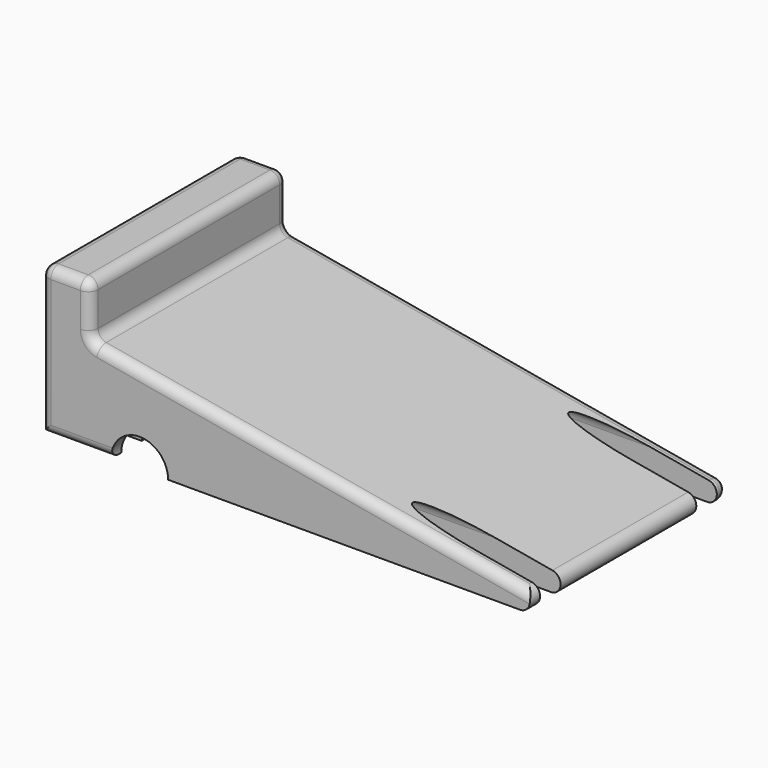
from build123d import *

# Parameters (mm, degrees)
F1_DEPTH = 15.875
F3_DEPTH = 76.201
F5_DEPTH = 31.751
F6_F1_R  = 1.27
F6_F2_R  = 1.27


with BuildPart() as f1:
    # F0 (on Front) → F1 (new body, symmetric)
    with BuildSketch(Plane.XZ):
        Polygon((-38.1, 19.05), (-38.1, 0), (38.1, 0), (-31.75, 12.3164396025), (-31.75, 19.05), align=None)
    extrude(amount=F1_DEPTH, both=True)

    # F2 (on face) → F3 (cut, through all)
    with BuildSketch(Plane(origin=(-38.1, 0, 0), x_dir=(0, -1, 0), z_dir=(-1, 0, 0))):
        with BuildLine():
            Line((-10.922, 0), (-10.922, 3.81))
            ThreePointArc((-10.922, 3.81), (-12.5728756711, 5.4608756711), (-14.2237513422, 3.81))
            Line((-14.2237513422, 3.81), (-14.2237513422, 0))
            Line((-14.2237513422, 0), (-10.922, 0))
        make_face()
        with BuildLine():
            Line((14.2237513422, 0), (14.2237513422, 3.81))
            ThreePointArc((14.2237513422, 3.81), (12.5728756711, 5.4608756711), (10.922, 3.81))
            Line((10.922, 3.81), (10.922, 0))
            Line((10.922, 0), (14.2237513422, 0))
        make_face()
    extrude(amount=-F3_DEPTH, mode=Mode.SUBTRACT)

    # F4 (on face) → F5 (cut, through all)
    with BuildSketch(Plane(origin=(0, 15.875, 0), x_dir=(-1, 0, 0), z_dir=(0, 1, 0))):
        with BuildLine():
            ThreePointArc((29.083, 0), (25.4, 3.683), (21.717, 0))
            Line((21.717, 0), (29.083, 0))
        make_face()
    extrude(amount=-F5_DEPTH, mode=Mode.SUBTRACT)

    # F6: fillet of radius 1.27 on 17 edges, made by hand

    # F6_f1
    f6_f1_edges = [f1.edges().sort_by_distance(p)[0] for p in [
        (-31.75, 0, 12.3164396025),
    ]]
    fillet(f6_f1_edges, radius=F6_F1_R)

    # F6_f2
    f6_f2_edges = [f1.edges().sort_by_distance(p)[0] for p in [
        (38.1, 0, 0),
        (38.1, 15.0493756711, 0),
        (38.1, -15.0493756711, 0),
        (-31.75, 0, 19.05),
        (-38.1, 0, 19.05),
        (-38.1, 15.0493756711, 0),
        (-38.1, 0, 0),
        (-33.5915, -15.875, 0),
        (8.1915, 15.875, 0),
        (-33.5915, 15.875, 0),
        (3.6997334072, -15.875, 6.0656951439),
        (-38.1, -15.875, 9.525),
        (-38.1, 15.875, 9.525),
        (-34.925, -15.875, 19.05),
        (-34.925, 15.875, 19.05),
        (3.6997334072, 15.875, 6.0656951439),
        (-31.4528764428, 15.875, 12.5657558698),
        (-31.4528764428, -15.875, 12.5657558698),
    ]]
    fillet(f6_f2_edges, radius=F6_F2_R)


solid = f1.part
